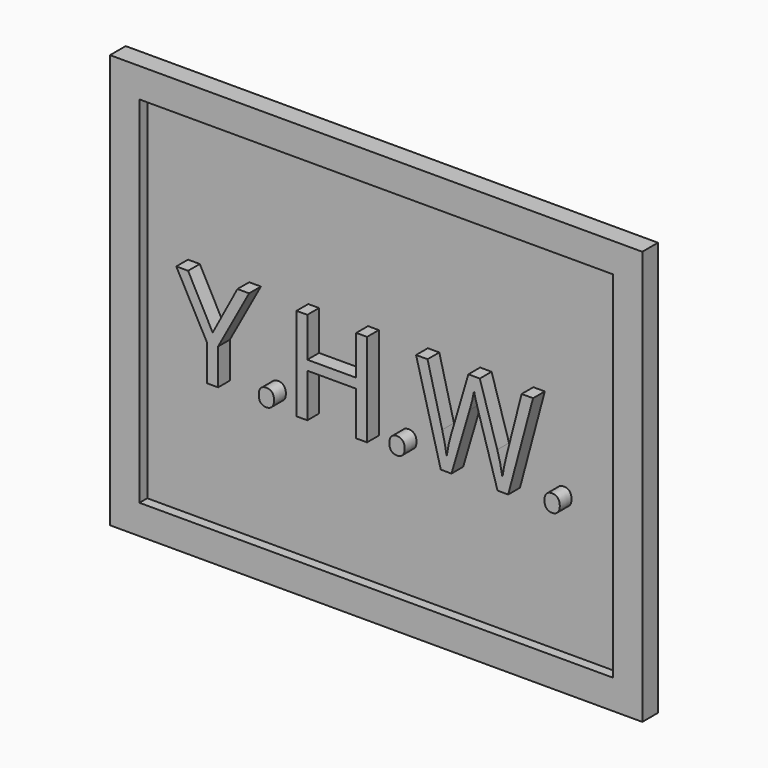
from build123d import *

# Parameters (mm, degrees)
F0_W         = 543.2
F0_H         = 422.4
F0_W_2       = 483.2
F0_H_2       = 362.4
F1_DEPTH     = 20
F2_DEPTH     = 10
F3_W         = 200
F3_H         = 100
F3_R         = 15
F4_DEPTH     = 15
F5_DEPTH     = 5
F6_TEXT_SIZE = 132.7800829876
F7_DEPTH     = 25


# Not quite as in the source:
# - Text() gives the source's letters only with a copy of the font that has no kerning and outlines rounded to 1/6400 em; it was checked with that copy


with BuildPart() as f1:
    # F0 (on Front) → F1 (new body)
    with BuildSketch(Plane.XZ):
        Rectangle(F0_W, F0_H)
        Rectangle(F0_W_2, F0_H_2, mode=Mode.SUBTRACT)
    extrude(amount=F1_DEPTH)

    # F0 (on Front) → F2 (join)
    with BuildSketch(Plane.XZ):
        Rectangle(F0_W_2, F0_H_2)
    extrude(amount=F2_DEPTH)

    # F3 (on face) → F4 (join)
    with BuildSketch(Plane.XZ):
        Rectangle(F3_W, F3_H)
        Circle(F3_R, mode=Mode.SUBTRACT)
    extrude(amount=-F4_DEPTH)

    # F3 (on face) → F5 (join)
    with BuildSketch(Plane.XZ):
        Circle(F3_R)
    extrude(amount=-F5_DEPTH)

    # F6 (on Front) → F7 (join)
    with BuildSketch(Plane.XZ):
        with Locations((-200, -48.0830861811)):
            Text('Y.H.W.', F6_TEXT_SIZE, font='Open Sans', text_align=(TextAlign.LEFT, TextAlign.BOTTOM))
    extrude(amount=F7_DEPTH)


solid = f1.part
